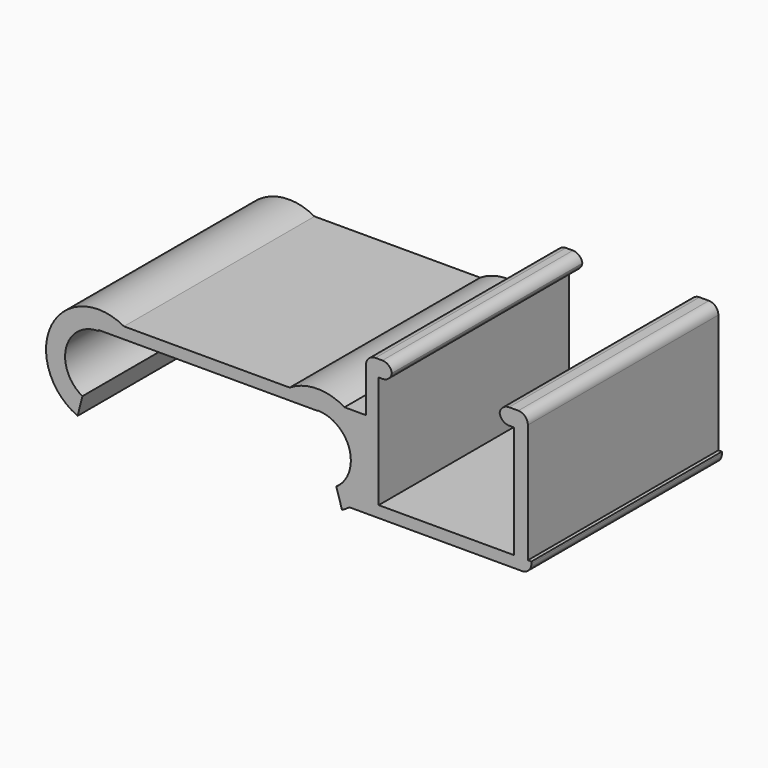
from build123d import *

# Parameters (mm, degrees)
F0_W        = 23
F0_H        = 25
F1_DEPTH    = 1.2
F3_DEPTH    = 25
F5_W        = 1.3906080276
F5_H        = 1.7
F5_W_2      = 1.5159434646
F6_DEPTH    = 25
F7_T1_DEPTH = 30


# Not quite as in the source:
# - a fillet or chamfer that OpenCascade refuses, or shapes differently, is made with other operations: its cross-section is extruded or revolved along the edge and cut away or added


with BuildPart() as f1:
    # F0 (on Top) → F1 (new body)
    with BuildSketch(Plane.XY):
        Rectangle(F0_W, F0_H)
    extrude(amount=F1_DEPTH)

    # F2 (on face) → F3 (join)
    with BuildSketch(Plane.XZ.offset(12.5)):
        with BuildLine():
            ThreePointArc((-8.8198933508, 1.2), (-16.4322899898, -1.1691927474), (-13.6809007153, -8.6519404997))
            Line((-13.6809007153, -8.6519404997), (-13.1818733439, -6.6722285874))
            ThreePointArc((-13.1818733439, -6.6722285874), (-14.8938387487, -2.747327312), (-11.5259407878, -0.1029107612))
            Line((-11.5259407878, -0.1029107612), (-11.5, 0))
            Line((-11.5, 0), (-11.5, 1.2))
            Line((-11.5, 1.2), (-8.8198933508, 1.2))
        make_face()
        with BuildLine():
            ThreePointArc((17, -3.4602172673), (14.1631160155, 1.3520392811), (8.578977059, 1.2))
            Line((8.578977059, 1.2), (11.5, 1.2))
            Line((11.5, 1.2), (11.5, 0.0397827327))
            ThreePointArc((11.5, 0.0397827327), (13.9748737342, -0.9853435331), (15, -3.4602172673))
            ThreePointArc((15, -3.4602172673), (14.5929628971, -5.0983810311), (13.4665254188, -6.3555199764))
            Line((13.4665254188, -6.3555199764), (14.0745145934, -8.3204512748))
            ThreePointArc((14.0745145934, -8.3204512748), (16.2122091562, -6.2966031487), (17, -3.4602172673))
        make_face()
    extrude(amount=-F3_DEPTH)

    # F5 (on face) → F6 (join)
    with BuildSketch(Plane.XZ.offset(12.5)):
        with Locations((18.6200318858, 6.0247716144)):
            Rectangle(F5_W, F5_H)
        with BuildLine():
            ThreePointArc((16.5864266455, -1.367787106), (17, -3.4602172673), (16.5864266455, -5.5526474285))
            Line((16.5864266455, -5.5526474285), (16.5864266455, -6.6252283856))
            Line((16.5864266455, -6.6252283856), (17.924727872, -6.6252283856))
            Line((17.924727872, -6.6252283856), (17.924727872, 5.1747716144))
            Line((17.924727872, 5.1747716144), (17.924727872, 6.8747716144))
            Line((17.924727872, 6.8747716144), (16.5864266455, 6.8747716144))
            Line((16.5864266455, 6.8747716144), (16.5864266455, 1.253477479))
            Line((16.5864266455, 1.253477479), (16.5864266455, -1.367787106))
        make_face()
        Polygon((32.124727872, -6.6252283856), (33.5864266455, -6.6252283856), (33.5864266455, 6.8747716144), (32.124727872, 6.8747716144), (32.124727872, 5.1747716144), align=None)
        with Locations((31.3667561397, 6.0247716144)):
            Rectangle(F5_W_2, F5_H)
        with BuildLine():
            Line((14.8461437412, -7.8252283856), (16.5864266455, -7.8252283856))
            Line((16.5864266455, -7.8252283856), (33.9574068785, -7.8252283856))
            Line((33.9574068785, -7.8252283856), (33.9574068785, -6.6252283856))
            Line((33.9574068785, -6.6252283856), (33.5864266455, -6.6252283856))
            Line((33.5864266455, -6.6252283856), (32.124727872, -6.6252283856))
            Line((32.124727872, -6.6252283856), (17.924727872, -6.6252283856))
            Line((17.924727872, -6.6252283856), (16.5864266455, -6.6252283856))
            Line((16.5864266455, -6.6252283856), (16.5864266455, -5.5526474285))
            ThreePointArc((16.5864266455, -5.5526474285), (15.8667169456, -6.8041345983), (14.8461437412, -7.8252283856))
        make_face()
        with BuildLine():
            ThreePointArc((14.333916343, 1.253477479), (15.6714164585, 0.1243726298), (16.5864266455, -1.367787106))
            Line((16.5864266455, -1.367787106), (16.5864266455, 1.253477479))
            Line((16.5864266455, 1.253477479), (14.333916343, 1.253477479))
        make_face()
    extrude(amount=-F6_DEPTH)

    # F7: fillet of radius 1 on 7 edges, made by hand

    # F7_s2 → F7_t1 (cut)
    with BuildSketch(Plane.XZ.offset(-15)):
        with BuildLine():
            ThreePointArc((33.5864266455, 5.8747716144), (33.2935334267, 6.5818783956), (32.5864266455, 6.8747716144))
            Line((32.5864266455, 6.8747716144), (33.5864266455, 6.8747716144))
            Line((33.5864266455, 6.8747716144), (33.5864266455, 5.8747716144))
        make_face()
        with BuildLine():
            ThreePointArc((17.5864266455, 6.8747716144), (16.8793198643, 6.5818783956), (16.5864266455, 5.8747716144))
            Line((16.5864266455, 5.8747716144), (16.5864266455, 6.8747716144))
            Line((16.5864266455, 6.8747716144), (17.5864266455, 6.8747716144))
        make_face()
        with BuildLine():
            ThreePointArc((18.3153358996, 5.1747716144), (19.0224426808, 5.4676648332), (19.3153358996, 6.1747716144))
            Line((19.3153358996, 6.1747716144), (19.3153358996, 5.1747716144))
            Line((19.3153358996, 5.1747716144), (18.3153358996, 5.1747716144))
        make_face()
        with BuildLine():
            ThreePointArc((30.6087844074, 6.1747716144), (30.9016776262, 5.4676648332), (31.6087844074, 5.1747716144))
            Line((31.6087844074, 5.1747716144), (30.6087844074, 5.1747716144))
            Line((30.6087844074, 5.1747716144), (30.6087844074, 6.1747716144))
        make_face()
        with BuildLine():
            ThreePointArc((31.6087844074, 6.8747716144), (30.9016776262, 6.5818783956), (30.6087844074, 5.8747716144))
            Line((30.6087844074, 5.8747716144), (30.6087844074, 6.8747716144))
            Line((30.6087844074, 6.8747716144), (31.6087844074, 6.8747716144))
        make_face()
        with BuildLine():
            ThreePointArc((18.3153358996, 6.8747716144), (19.0224426808, 6.5818783956), (19.3153358996, 5.8747716144))
            Line((19.3153358996, 5.8747716144), (19.3153358996, 6.8747716144))
            Line((19.3153358996, 6.8747716144), (18.3153358996, 6.8747716144))
        make_face()
        with BuildLine():
            ThreePointArc((32.9574068785, -7.8252283856), (33.6645136597, -7.5323351668), (33.9574068785, -6.8252283856))
            Line((33.9574068785, -6.8252283856), (33.9574068785, -7.8252283856))
            Line((33.9574068785, -7.8252283856), (32.9574068785, -7.8252283856))
        make_face()
    extrude(amount=F7_T1_DEPTH, mode=Mode.SUBTRACT)


solid = f1.part
